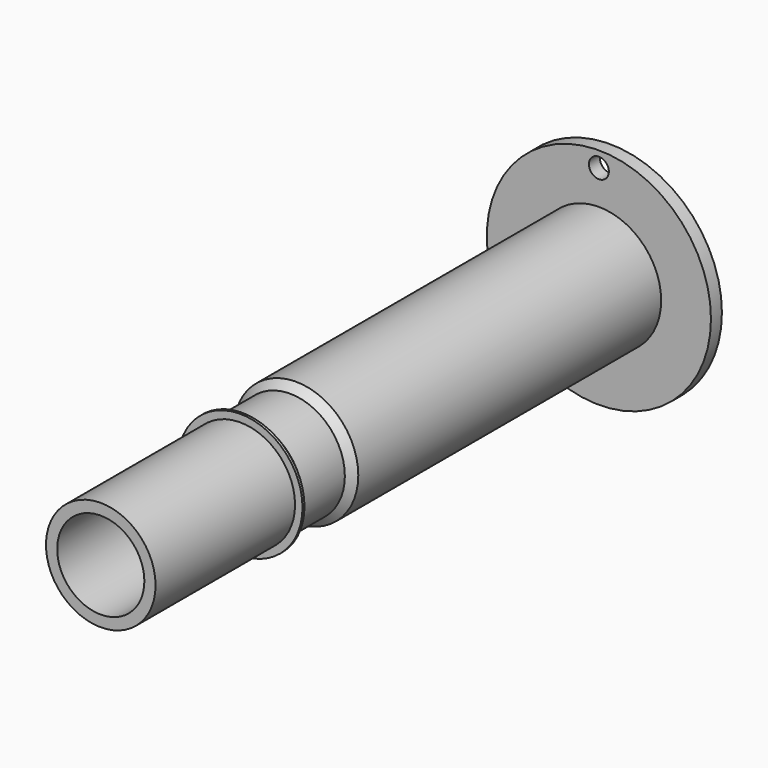
from build123d import *

# Parameters (mm, degrees)
F0_R      = 90
F0_R_2    = 8
F1_DEPTH  = 11
F2_R      = 50
F3_DEPTH  = 310
F4_R      = 44
F5_DEPTH  = 190
F6_R      = 35
F7_DEPTH  = 350
F8_SIZE   = 5.99999
F10_R     = 50
F11_DEPTH = 8
F12_SIZE  = 5.99999


# Not quite as in the source:
# - a fillet or chamfer is up to 0.001 mm smaller than in the source, because OpenCascade refuses the exact size


with BuildPart() as f1:
    # F0 (on Front) → F1 (new body)
    with BuildSketch(Plane.XZ):
        Circle(F0_R)
        with Locations((0, 77.5)):
            Circle(F0_R_2, mode=Mode.SUBTRACT)
    extrude(amount=F1_DEPTH)

    # F2 (on face) → F3 (join)
    with BuildSketch(Plane.XZ.offset(11)):
        Circle(F2_R)
    extrude(amount=F3_DEPTH)

    # F4 (on face) → F5 (join)
    with BuildSketch(Plane.XZ.offset(321)):
        Circle(F4_R)
    extrude(amount=F5_DEPTH)

    # F6 (on face) → F7 (cut)
    with BuildSketch(Plane.XZ.offset(511)):
        Circle(F6_R)
    extrude(amount=-F7_DEPTH, mode=Mode.SUBTRACT)

    # F8 (size 6 in the source; OpenCascade refuses exactly that, so slightly less here)
    f8_edges = [f1.edges().sort_by_distance(p)[0] for p in [
        (-50, -321, 0),
    ]]
    chamfer(f8_edges, length=F8_SIZE)

    # F10 (on offset) → F11 (join)
    with BuildSketch(Plane.XZ.offset(371)):
        Circle(F10_R)
    extrude(amount=-F11_DEPTH)

    # F12 (size 6 in the source; OpenCascade refuses exactly that, so slightly less here)
    f12_edges = [f1.edges().sort_by_distance(p)[0] for p in [
        (-50, -363, 0),
    ]]
    chamfer(f12_edges, length=F12_SIZE)


solid = f1.part
